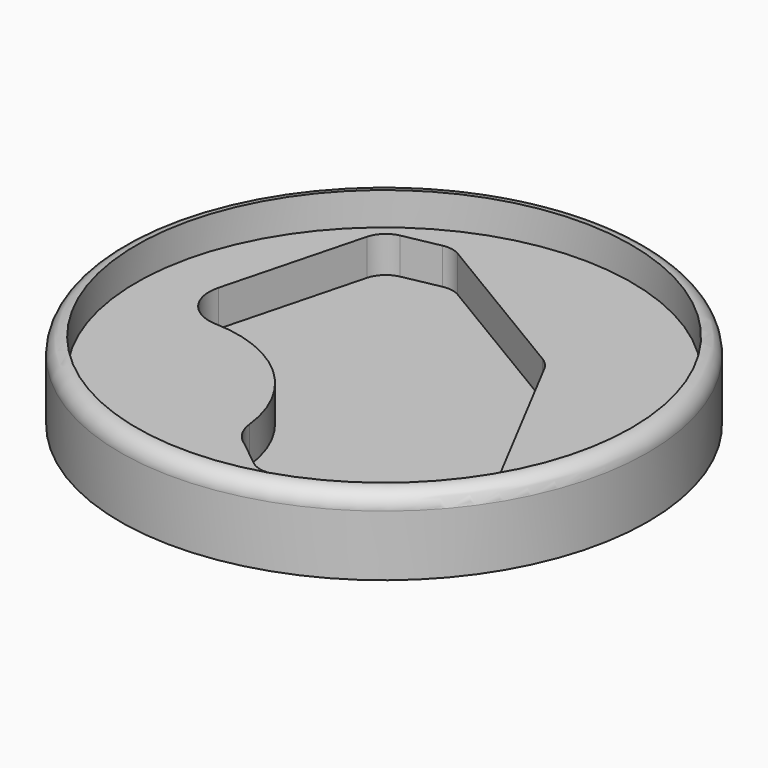
from build123d import *

# Parameters (mm, degrees)
F0_R     = 16.05
F1_DEPTH = 2.7
F2_R     = 16.05
F2_R_2   = 15.05
F3_DEPTH = 2
F4_R     = 0.99999
F5_R     = 16.05
F6_DEPTH = 0.5


# Not quite as in the source:
# - a fillet or chamfer is up to 0.001 mm smaller than in the source, because OpenCascade refuses the exact size


with BuildPart() as f1:
    # F0 (on Top) → F1 (new body)
    with BuildSketch(Plane.XY):
        Circle(F0_R)
        with BuildLine():
            ThreePointArc((-0.6780739779, -9.7725818409), (-1.4027582732, -9.0367076796), (-1.7421252674, -8.061254886))
            ThreePointArc((-1.7421252674, -8.061254886), (-4.3074337596, -3.0577956653), (-9.536973063, -0.9920438631))
            ThreePointArc((-9.536973063, -0.9920438631), (-11.3022646183, -0.0029612607), (-11.6691612698, 1.9869948988))
            Line((-11.6691612698, 1.9869948988), (-9.4391799782, 10.4875703743))
            ThreePointArc((-9.4391799782, 10.4875703743), (-9.0171024282, 11.1985139757), (-8.2824484024, 11.5778208766))
            Line((-8.2824484024, 11.5778208766), (-6.0604061806, 12.0222295772))
            ThreePointArc((-6.0604061806, 12.0222295772), (-5.5105978167, 12.029415178), (-4.9951399441, 11.8379888177))
            Line((-4.9951399441, 11.8379888177), (4.893855989, 5.9114030387))
            ThreePointArc((4.893855989, 5.9114030387), (5.3199805506, 5.5689093688), (5.6374422976, 5.1238227536))
            Line((5.6374422976, 5.1238227536), (12.1259901628, -7.2648903372))
            ThreePointArc((12.1259901628, -7.2648903372), (12.1554437407, -8.5973863607), (11.1125476049, -9.4273145597))
            Line((11.1125476049, -9.4273145597), (2.1831787086, -11.347409045))
            ThreePointArc((2.1831787086, -11.347409045), (1.5325569034, -11.3429782119), (0.9450171886, -11.0634689113))
            Line((0.9450171886, -11.0634689113), (-0.6780739779, -9.7725818409))
        make_face(mode=Mode.SUBTRACT)
    extrude(amount=F1_DEPTH)

    # F2 (on face) → F3 (join)
    with BuildSketch(Plane.XY.offset(2.7)):
        Circle(F2_R)
        Circle(F2_R_2, mode=Mode.SUBTRACT)
    extrude(amount=F3_DEPTH)

    # F4 (radius 1 in the source; OpenCascade refuses exactly that, so slightly less here)
    f4_edges = [f1.edges().sort_by_distance(p)[0] for p in [
        (-16.05, 0, 4.7),
    ]]
    fillet(f4_edges, radius=F4_R)

    # F5 (on face) → F6 (join)
    with BuildSketch(Plane.XY):
        Circle(F5_R)
    extrude(amount=F6_DEPTH)


solid = f1.part
